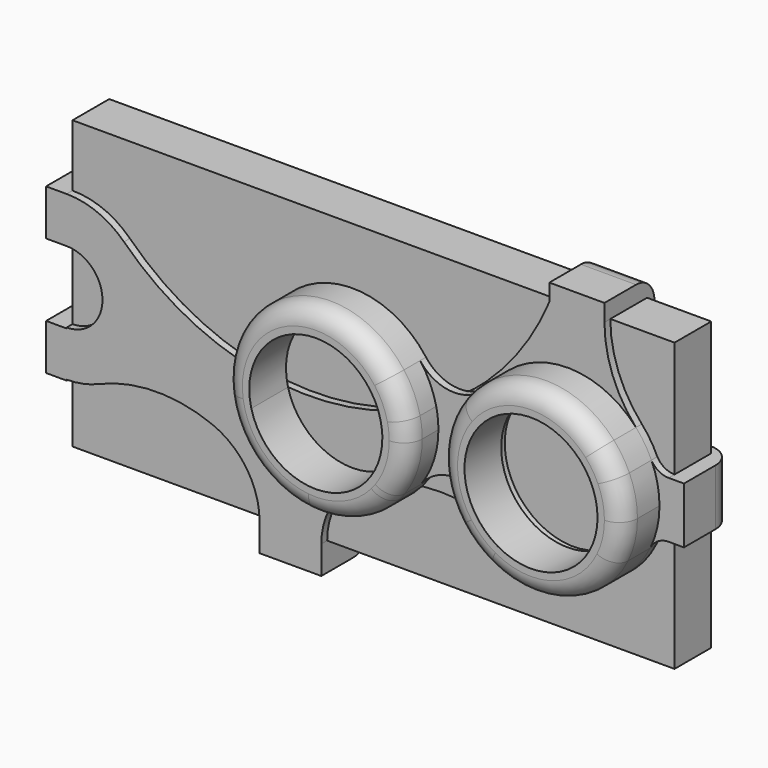
from build123d import *

# Parameters (mm, degrees)
F0_W      = 166.624
F0_H      = 79.502
F1_DEPTH  = 12.7
F3_R      = 19.05
F3_W      = 15.2498179367
F3_H      = 4.727289783
F3_W_2    = 4.2314800982
F3_H_2    = 15.5652722449
F3_W_3    = 17.0839390975
F3_H_3    = 7.7993963947
F3_W_4    = 5.6899759536
F3_H_4    = 12.7
F4_DEPTH  = 2.032
F5_DEPTH  = 15.24
F7_DEPTH  = 15.2498179367
F9_DEPTH  = 15.5652722449
F11_DEPTH = 17.0839390975
F13_DEPTH = 12.7
F15_DEPTH = 12.7
F16_R     = 6.35
F18_DEPTH = 2.032
F17_R     = 19.05
F17_R_2   = 18.415
F19_DEPTH = 12.7
F20_R     = 5.08


# Not quite as in the source:
# - a feature of the source that left no trace in its solid (it failed there, or was rolled back) is left out


with BuildPart() as f1:
    # F0 (on Front) → F1 (new body)
    with BuildSketch(Plane.XZ):
        Rectangle(F0_W, F0_H)
    extrude(amount=F1_DEPTH)


with BuildPart() as f4:
    # F3 (on face) → F4 (new body)
    with BuildSketch(Plane.XZ.offset(12.7)):
        with BuildLine():
            Line((83.312, -7.9452722449), (83.312, 7.62))
            ThreePointArc((83.312, 7.62), (80.5537024075, 8.3652624791), (78.5460535381, 10.3982326679))
            ThreePointArc((78.5460535381, 10.3982326679), (76.662940796, 13.8512035585), (74.2693311981, 16.9720615598))
            ThreePointArc((74.2693311981, 16.9720615598), (67.7983810803, 27.5541815195), (65.5418179367, 39.751))
            Line((65.5418179367, 39.751), (50.292, 39.751))
            ThreePointArc((50.292, 39.751), (-2.2901946449, -3.3376030905), (-67.4321012743, 16.1058253792))
            ThreePointArc((-67.4321012743, 16.1058253792), (-74.7303608062, 20.9266400417), (-83.312, 22.6178866096))
            Line((-83.312, 22.6178866096), (-83.312, 9.9178866096))
            ThreePointArc((-83.312, 9.9178866096), (-73.3941133904, 0), (-83.312, -9.9178866096))
            Line((-83.312, -9.9178866096), (-83.312, -10.16))
            Line((-83.312, -10.16), (-83.312, -22.6178866096))
            ThreePointArc((-83.312, -22.6178866096), (-78.7711442585, -22.1573785413), (-74.4151953336, -20.7946065463))
            ThreePointArc((-74.4151953336, -20.7946065463), (-58.7402465196, -17.4860386913), (-42.9917926654, -20.424889278))
            ThreePointArc((-42.9917926654, -20.424889278), (-33.4884475886, -28.0825335776), (-29.9107422883, -39.751))
            Line((-29.9107422883, -39.751), (-12.8268031908, -39.751))
            ThreePointArc((-12.8268031908, -39.751), (-10.0533012351, -29.573156585), (-2.4996713636, -22.2094967991))
            ThreePointArc((-2.4996713636, -22.2094967991), (20.2738138752, -16.3141101101), (43.0472991139, -22.2094967991))
            ThreePointArc((43.0472991139, -22.2094967991), (63.0016110107, -24.2270310981), (78.1990053344, -11.1394715972))
            ThreePointArc((78.1990053344, -11.1394715972), (80.2976334018, -8.8094548883), (83.312, -7.9452722449))
        make_face()
        with Locations((55.372, 0)):
            Circle(F3_R, mode=Mode.SUBTRACT)
        with Locations((57.9169089684, 42.1146448915)):
            Rectangle(F3_W, F3_H)
        with Locations((85.4277400491, -0.1626361225)):
            Rectangle(F3_W_2, F3_H_2)
        with Locations((-21.3687727395, -43.6506981973)):
            Rectangle(F3_W_3, F3_H_3)
        Polygon((-89.0019759536, -22.86), (-83.312, -22.86), (-83.312, -22.6178866096), (-83.312, -10.16), (-89.0019759536, -10.16), align=None)
        with Locations((-86.1569879768, 16.2678866096)):
            Rectangle(F3_W_4, F3_H_4)
    extrude(amount=F4_DEPTH)

    # F3 (on face) → F5 (join)
    with BuildSketch(Plane.XZ.offset(12.7)):
        Polygon((-89.0019759536, -22.86), (-83.312, -22.86), (-83.312, -22.6178866096), (-83.312, -10.16), (-89.0019759536, -10.16), align=None)
        with Locations((-86.1569879768, 16.2678866096)):
            Rectangle(F3_W_4, F3_H_4)
        with Locations((-21.3687727395, -43.6506981973)):
            Rectangle(F3_W_3, F3_H_3)
        with Locations((57.9169089684, 42.1146448915)):
            Rectangle(F3_W, F3_H)
        with Locations((85.4277400491, -0.1626361225)):
            Rectangle(F3_W_2, F3_H_2)
    extrude(amount=-F5_DEPTH)

    # F6 (on face) → F7 (join, through all)
    with BuildSketch(Plane.YZ.offset(65.5418179367)):
        with BuildLine():
            add(Edge.make_bspline(
                [(2.54, 37.211), (1.2037418783, 37.2195914388), (2.2650531027, 38.99884969), (-5.08, 39.751)],
                knots=[0, 0, 0, 0, 8.0321852568, 8.0321852568, 8.0321852568, 8.0321852568], degree=3))
            Line((2.54, 37.211), (2.54, 39.751))
            Line((2.54, 39.751), (-5.08, 39.751))
        make_face()
    extrude(amount=-F7_DEPTH)

    # F8 (on face) → F9 (join, through all)
    with BuildSketch(Plane(origin=(0, 0, -7.9452722449), x_dir=(1, 0, 0), z_dir=(0, 0, -1))):
        with BuildLine():
            add(Edge.make_bspline(
                [(80.772, -2.54), (80.7990506291, -0.8979742997), (82.3285877705, -2.1777907386), (83.312, 5.08)],
                knots=[0, 0, 0, 0, 8.0321852568, 8.0321852568, 8.0321852568, 8.0321852568], degree=3))
            Line((80.772, -2.54), (83.312, -2.54))
            Line((83.312, -2.54), (83.312, 5.08))
        make_face()
    extrude(amount=-F9_DEPTH)

    # F10 (on face) → F11 (join, through all)
    with BuildSketch(Plane(origin=(-29.9107422883, 0, 0), x_dir=(0, -1, 0), z_dir=(-1, 0, 0))):
        with BuildLine():
            add(Edge.make_bspline(
                [(-2.54, -37.211), (-1.2959121959, -37.1081680059), (-1.9826430362, -38.481), (5.08, -39.751)],
                knots=[0, 0, 0, 0, 8.0321852568, 8.0321852568, 8.0321852568, 8.0321852568], degree=3))
            Line((-2.54, -37.211), (-2.54, -39.751))
            Line((-2.54, -39.751), (5.08, -39.751))
        make_face()
    extrude(amount=-F11_DEPTH)

    # F12 (on face) → F13 (join, through all)
    with BuildSketch(Plane(origin=(0, 0, -22.86), x_dir=(1, 0, 0), z_dir=(0, 0, -1))):
        with BuildLine():
            Line((-83.312, -2.54), (-80.772, -2.54))
            add(Edge.make_bspline(
                [(-80.772, -2.54), (-80.6815177202, -1.0831034742), (-82.1486189961, -2.0507695153), (-83.312, 6.096)],
                knots=[0, 0, 0, 0, 9.0017829345, 9.0017829345, 9.0017829345, 9.0017829345], degree=3))
            Line((-83.312, 6.096), (-83.312, -2.54))
        make_face()
    extrude(amount=-F13_DEPTH)

    # F14 (on face) → F15 (join, through all)
    with BuildSketch(Plane.XY.offset(22.6178866096)):
        with BuildLine():
            add(Edge.make_bspline(
                [(-80.7734341134, 2.4546581032), (-80.8589532971, 1.342135598), (-82.2274386883, 1.9601618405), (-83.312, -4.8822709359)],
                knots=[0, 0, 0, 0, 7.7636875572, 7.7636875572, 7.7636875572, 7.7636875572], degree=3))
            Line((-80.7734341134, 2.4546581032), (-83.312, 2.54))
            Line((-83.312, 2.54), (-83.312, -4.7201365232))
            Line((-83.312, -4.7201365232), (-83.312, -4.8822709359))
        make_face()
    extrude(amount=-F15_DEPTH)

    # F16
    f16_edges = [f4.edges().sort_by_distance(p)[0] for p in [
        (-21.368773, 2.54, -47.550396),
        (-89.001976, 2.54, -16.51),
        (-89.001976, 2.54, 16.267887),
        (87.54348, 2.54, -0.162636),
        (57.916909, 2.54, 44.47829),
    ]]
    fillet(f16_edges, radius=F16_R)


with BuildPart() as f18:
    # F17 (on face) → F18 (new body)
    with BuildSketch(Plane.XZ.offset(14.732)):
        with BuildLine():
            ThreePointArc((28.2864236116, 10.7885061807), (24.5314617002, 8.0209659875), (20.6062090392, 5.5007657527))
            ThreePointArc((20.6062090392, 5.5007657527), (21.0578525442, 2.7668475206), (21.209, 0))
            ThreePointArc((21.209, 0), (19.9758983224, -7.8179936988), (16.3963208288, -14.876902268))
            ThreePointArc((16.3963208288, -14.876902268), (25.5905, -10.1773472949), (34.7846791712, -14.876902268))
            ThreePointArc((34.7846791712, -14.876902268), (29.972808178, 0.2026198097), (35.0246425652, 15.2034550488))
            ThreePointArc((35.0246425652, 15.2034550488), (32.0447675603, 12.4019200322), (28.2864236116, 10.7885061807))
        make_face()
        with BuildLine():
            ThreePointArc((16.1563574348, 15.2034550488), (18.8967351732, 10.5885071929), (20.6062090392, 5.5007657527))
            ThreePointArc((20.6062090392, 5.5007657527), (24.5314617002, 8.0209659875), (28.2864236116, 10.7885061807))
            ThreePointArc((28.2864236116, 10.7885061807), (21.5626169277, 11.1860010324), (16.1563574348, 15.2034550488))
        make_face()
    extrude(amount=F18_DEPTH)

    # F17 (on face) → F19 (join)
    with BuildSketch(Plane.XZ.offset(14.732)):
        with BuildLine():
            ThreePointArc((74.2693311981, 16.9720615598), (54.2284807525, 25.3742460722), (35.0246425652, 15.2034550488))
            ThreePointArc((35.0246425652, 15.2034550488), (29.972808178, 0.2026198097), (34.7846791712, -14.876902268))
            ThreePointArc((34.7846791712, -14.876902268), (38.5125210941, -18.99784122), (43.0472991139, -22.2094967991))
            ThreePointArc((43.0472991139, -22.2094967991), (63.0016110107, -24.2270310981), (78.1990053344, -11.1394715972))
            ThreePointArc((78.1990053344, -11.1394715972), (80.1203932357, -5.7163827945), (80.772, 0))
            ThreePointArc((80.772, 0), (80.209280043, 5.3169088827), (78.5460535381, 10.3982326679))
            ThreePointArc((78.5460535381, 10.3982326679), (76.662940796, 13.8512035585), (74.2693311981, 16.9720615598))
        make_face()
        with Locations((55.372, 0)):
            Circle(F17_R, mode=Mode.SUBTRACT)
        with Locations((55.372, 0)):
            Circle(F17_R)
        with Locations((55.372, 0)):
            Circle(F17_R_2, mode=Mode.SUBTRACT)
        with BuildLine():
            ThreePointArc((-22.0352595619, -4.5491346088), (-7.5002575265, 18.1152156935), (14.1091283255, 2.0536621604))
            ThreePointArc((14.1091283255, 2.0536621604), (17.4014337238, 3.6947258621), (20.6062090392, 5.5007657527))
            ThreePointArc((20.6062090392, 5.5007657527), (18.8967351732, 10.5885071929), (16.1563574348, 15.2034550488))
            ThreePointArc((16.1563574348, 15.2034550488), (-13.9039135762, 23.4695400437), (-29.3314617697, -3.6217650399))
            ThreePointArc((-29.3314617697, -3.6217650399), (-25.6951347151, -4.1780837077), (-22.0352595619, -4.5491346088))
        make_face()
        with BuildLine():
            ThreePointArc((14.1091283255, 2.0536621604), (14.1952596538, 1.0284361636), (14.224, 0))
            ThreePointArc((14.224, 0), (-1.8986011289, -18.2717577812), (-22.0352595619, -4.5491346088))
            ThreePointArc((-22.0352595619, -4.5491346088), (-25.6951347151, -4.1780837077), (-29.3314617697, -3.6217650399))
            ThreePointArc((-29.3314617697, -3.6217650399), (-21.7360818632, -18.3665484622), (-6.6594189467, -25.2797727028))
            ThreePointArc((-6.6594189467, -25.2797727028), (-4.678865898, -23.6100705511), (-2.4996713636, -22.2094967991))
            ThreePointArc((-2.4996713636, -22.2094967991), (5.9863881024, -18.5416288768), (15.0267873519, -16.6083307198))
            ThreePointArc((15.0267873519, -16.6083307198), (15.7303734577, -15.7575023262), (16.3963208288, -14.876902268))
            ThreePointArc((16.3963208288, -14.876902268), (19.9758983224, -7.8179936988), (21.209, 0))
            ThreePointArc((21.209, 0), (21.0578525442, 2.7668475206), (20.6062090392, 5.5007657527))
            ThreePointArc((20.6062090392, 5.5007657527), (17.4014337238, 3.6947258621), (14.1091283255, 2.0536621604))
        make_face()
        with BuildLine():
            ThreePointArc((-2.4996713636, -22.2094967991), (-4.678865898, -23.6100705511), (-6.6594189467, -25.2797727028))
            ThreePointArc((-6.6594189467, -25.2797727028), (5.2394725231, -23.5844480112), (15.0267873519, -16.6083307198))
            ThreePointArc((15.0267873519, -16.6083307198), (5.9863881024, -18.5416288768), (-2.4996713636, -22.2094967991))
        make_face()
    extrude(amount=F19_DEPTH)

    # F20
    f20_edges = [f18.edges().sort_by_distance(p)[0] for p in [
        (32.197946, -27.432, -10.398233),
        (-1.722581, -27.432, 25.279773),
    ]]
    fillet(f20_edges, radius=F20_R)


solid = Compound([f1.part, f4.part, f18.part])
